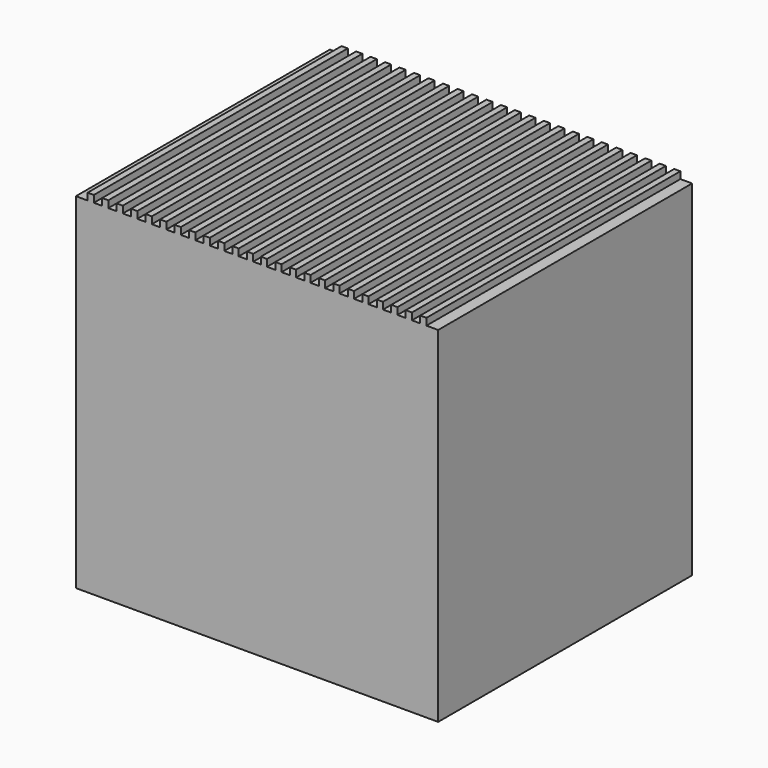
from build123d import *

# Parameters (mm, degrees)
F2_W         = 10.5
F2_H         = 9.2
F3_DEPTH     = 10
F4_W         = 0.18
F4_H         = 9.2
F5_DEPTH     = 0.2
F6_DEPTH     = 0.2
F7_TEXT_SIZE = 10.4738557841
F8_DEPTH     = 2


# Not quite as in the source:
# - Text() gives the source's letters only with a copy of the font that has no kerning and outlines rounded to 1/6400 em; it was checked with that copy


with BuildPart() as f3:
    # F2 (on Top) → F3 (new body)
    with BuildSketch(Plane.XY):
        Rectangle(F2_W, F2_H)
    extrude(amount=F3_DEPTH)

    # F4 (on face) → F5 (join)
    with BuildSketch(Plane.XY.offset(10)):
        with Locations((0.2, 0)):
            Rectangle(F4_W, F4_H)
        with Locations((0.62, 0)):
            Rectangle(F4_W, F4_H)
        with Locations((-0.2, 0)):
            Rectangle(F4_W, F4_H)
        with Locations((1.04, 0)):
            Rectangle(F4_W, F4_H)
        with Locations((1.46, 0)):
            Rectangle(F4_W, F4_H)
        with Locations((1.88, 0)):
            Rectangle(F4_W, F4_H)
        with Locations((2.3, 0)):
            Rectangle(F4_W, F4_H)
        with Locations((2.72, 0)):
            Rectangle(F4_W, F4_H)
        with Locations((3.14, 0)):
            Rectangle(F4_W, F4_H)
        with Locations((3.56, 0)):
            Rectangle(F4_W, F4_H)
        with Locations((3.98, 0)):
            Rectangle(F4_W, F4_H)
        with Locations((4.4, 0)):
            Rectangle(F4_W, F4_H)
        with Locations((4.82, 0)):
            Rectangle(F4_W, F4_H)
        with Locations((-4.82, 0)):
            Rectangle(F4_W, F4_H)
        with Locations((-3.98, 0)):
            Rectangle(F4_W, F4_H)
        with Locations((-4.4, 0)):
            Rectangle(F4_W, F4_H)
        with Locations((-2.72, 0)):
            Rectangle(F4_W, F4_H)
        with Locations((-1.88, 0)):
            Rectangle(F4_W, F4_H)
        with Locations((-2.3, 0)):
            Rectangle(F4_W, F4_H)
        with Locations((-1.04, 0)):
            Rectangle(F4_W, F4_H)
        with Locations((-3.56, 0)):
            Rectangle(F4_W, F4_H)
        with Locations((-0.62, 0)):
            Rectangle(F4_W, F4_H)
        with Locations((-3.14, 0)):
            Rectangle(F4_W, F4_H)
        with Locations((-1.46, 0)):
            Rectangle(F4_W, F4_H)
    extrude(amount=F5_DEPTH)

    # F4 (on face) → F6 (join)
    with BuildSketch(Plane.XY.offset(10)):
        with Locations((0.2, 0)):
            Rectangle(F4_W, F4_H)
        with Locations((0.62, 0)):
            Rectangle(F4_W, F4_H)
        with Locations((-0.2, 0)):
            Rectangle(F4_W, F4_H)
        with Locations((1.04, 0)):
            Rectangle(F4_W, F4_H)
        with Locations((1.46, 0)):
            Rectangle(F4_W, F4_H)
        with Locations((1.88, 0)):
            Rectangle(F4_W, F4_H)
        with Locations((2.3, 0)):
            Rectangle(F4_W, F4_H)
        with Locations((2.72, 0)):
            Rectangle(F4_W, F4_H)
        with Locations((3.14, 0)):
            Rectangle(F4_W, F4_H)
        with Locations((3.56, 0)):
            Rectangle(F4_W, F4_H)
        with Locations((3.98, 0)):
            Rectangle(F4_W, F4_H)
        with Locations((4.4, 0)):
            Rectangle(F4_W, F4_H)
        with Locations((4.82, 0)):
            Rectangle(F4_W, F4_H)
        with Locations((-4.82, 0)):
            Rectangle(F4_W, F4_H)
        with Locations((-3.98, 0)):
            Rectangle(F4_W, F4_H)
        with Locations((-4.4, 0)):
            Rectangle(F4_W, F4_H)
        with Locations((-2.72, 0)):
            Rectangle(F4_W, F4_H)
        with Locations((-1.88, 0)):
            Rectangle(F4_W, F4_H)
        with Locations((-2.3, 0)):
            Rectangle(F4_W, F4_H)
        with Locations((-1.04, 0)):
            Rectangle(F4_W, F4_H)
        with Locations((-3.56, 0)):
            Rectangle(F4_W, F4_H)
        with Locations((-0.62, 0)):
            Rectangle(F4_W, F4_H)
        with Locations((-3.14, 0)):
            Rectangle(F4_W, F4_H)
        with Locations((-1.46, 0)):
            Rectangle(F4_W, F4_H)
    extrude(amount=F6_DEPTH)

    # F7 (on face) → F8 (cut)
    with BuildSketch(Plane(origin=(0, 0, 0), x_dir=(1, 0, 0), z_dir=(0, 0, -1))):
        with Locations((-2.9415762983, -3.7507091183)):
            Text('2', F7_TEXT_SIZE, font='Open Sans', font_style=FontStyle.BOLD, text_align=(TextAlign.LEFT, TextAlign.BOTTOM))
    extrude(amount=-F8_DEPTH, mode=Mode.SUBTRACT)


solid = f3.part
